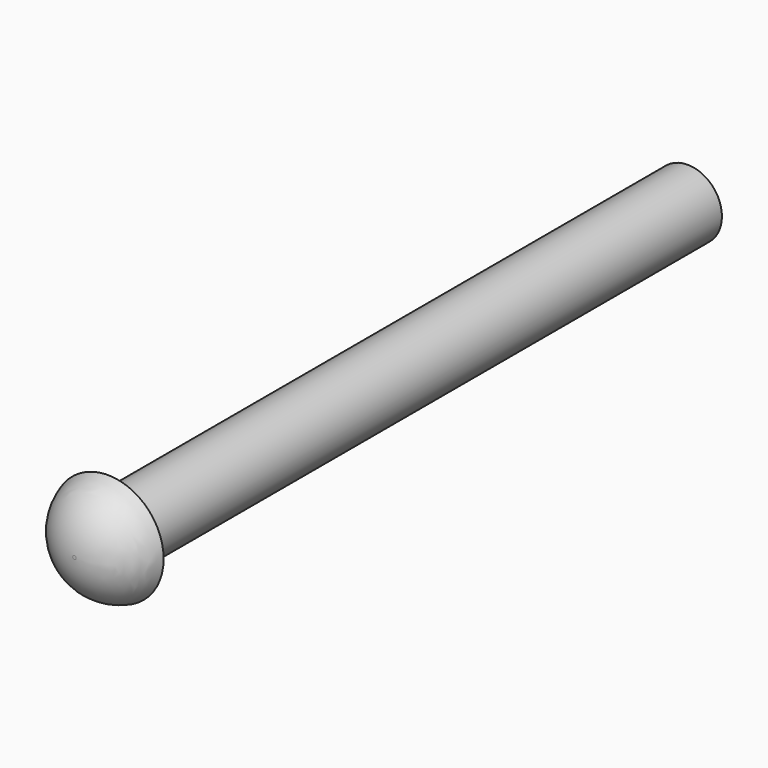
from build123d import *

# Parameters (mm, degrees)
F0_R     = 1.5621
F1_DEPTH = 33.02
F2_R     = 2.54
F3_DEPTH = 1.905


# Not quite as in the source:
# - a fillet or chamfer that OpenCascade refuses, or shapes differently, is made with other operations: its cross-section is extruded or revolved along the edge and cut away or added


with BuildPart() as f1:
    # F0 (on Front) → F1 (new body)
    with BuildSketch(Plane.XZ):
        with Locations((10.1929502562, 6.33663591)):
            Circle(F0_R)
    extrude(amount=F1_DEPTH)

    # F2 (on face) → F3 (join)
    with BuildSketch(Plane.XZ.offset(33.02)):
        with Locations((10.1929502562, 6.33663591)):
            Circle(F2_R)
    extrude(amount=F3_DEPTH)

    # F4: fillet of radius 2.54 on 1 edges, made by hand

    # F4_s1 → F4_t2 (revolve, cut)
    with BuildSketch(Plane.XY.offset(6.33663591)):
        with BuildLine():
            ThreePointArc((12.7329502562, -33.02), (11.829031818, -34.3930463142), (10.2736058313, -34.925))
            Line((10.2736058313, -34.925), (12.7329502562, -34.925))
            Line((12.7329502562, -34.925), (12.7329502562, -33.02))
        make_face()
    revolve(axis=Axis((10.1929502562, -34.925, 6.33663591), (0, -1, 0)), mode=Mode.SUBTRACT)


solid = f1.part
